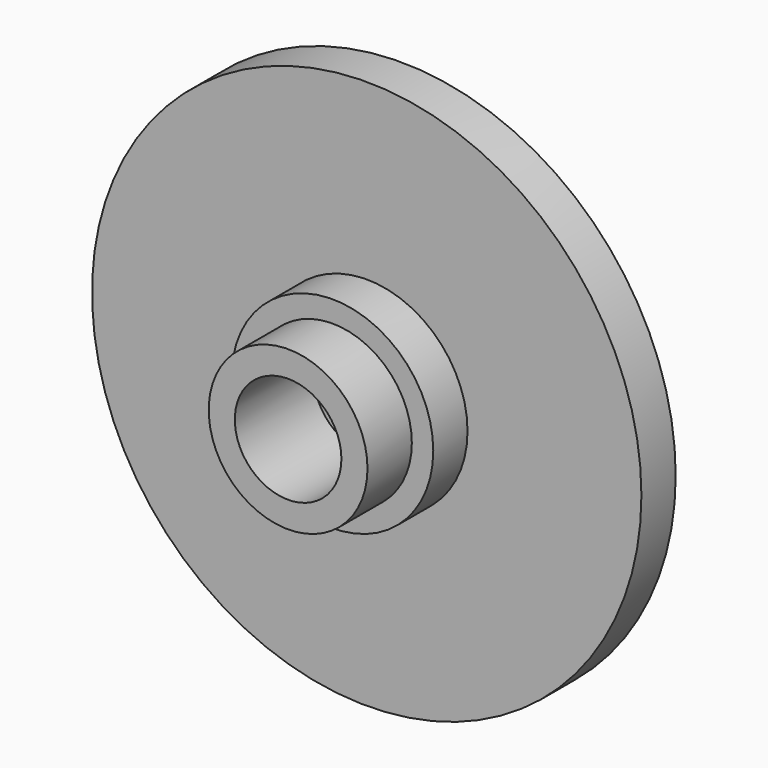
from build123d import *

# Parameters (mm, degrees)
F0_R     = 10.9
F0_R_2   = 4
F1_DEPTH = 1.7
F0_R_3   = 2.115
F0_R_4   = 3.15
F2_DEPTH = 3.4
F3_DEPTH = 5.6


with BuildPart() as f1:
    # F0 (on Front) → F1 (new body)
    with BuildSketch(Plane.XZ):
        Circle(F0_R)
        Circle(F0_R_2, mode=Mode.SUBTRACT)
    extrude(amount=F1_DEPTH)


with BuildPart() as f1b:
    # F0 (on Front) → F1, piece 2 (new body)
    with BuildSketch(Plane.XZ):
        Circle(F0_R_3)
    extrude(amount=F1_DEPTH)


with BuildPart() as f2:
    # F0 (on Front) → F2 (new body)
    with BuildSketch(Plane.XZ):
        Circle(F0_R_2)
        Circle(F0_R_4, mode=Mode.SUBTRACT)
    extrude(amount=F2_DEPTH)

    # F0 (on Front) → F3 (join)
    with BuildSketch(Plane.XZ):
        Circle(F0_R_4)
        Circle(F0_R_3, mode=Mode.SUBTRACT)
    extrude(amount=F3_DEPTH)


solid = Compound([f1.part, f1b.part, f2.part])
